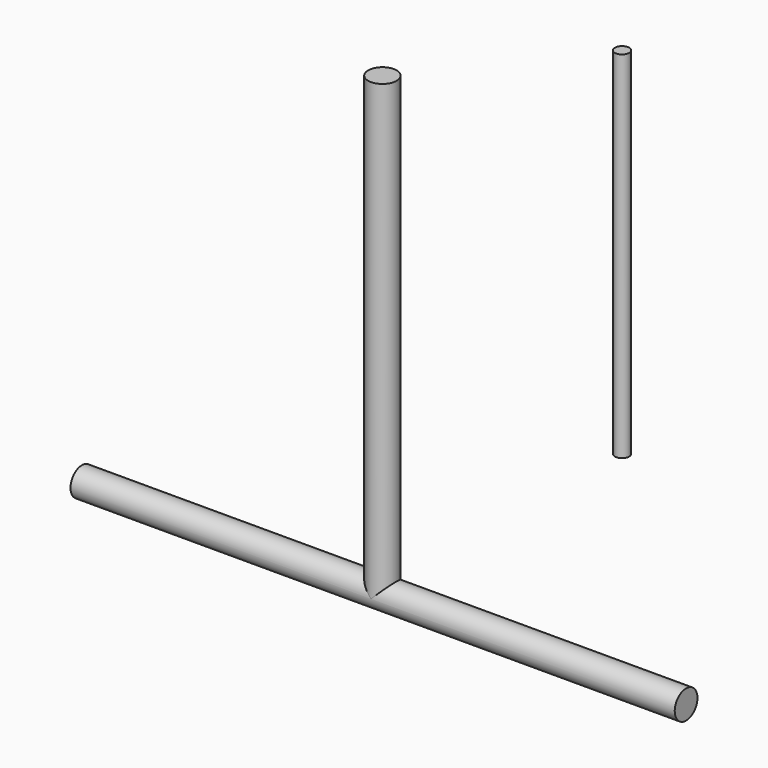
from build123d import *

# Parameters (mm, degrees)
F0_W     = 2.54
F0_H     = 81.28
F7_R     = 1.27
F8_DEPTH = 63.5


# Not quite as in the source:
# - the program builds the solid bodies; features that only make, move or delete a surface that nothing else refers to are left out


with BuildPart() as f1:
    # F0 (on Front) → F1 (revolve)
    with BuildSketch(Plane.XZ):
        with Locations((1.27, 0)):
            Rectangle(F0_W, F0_H)
    revolve(axis=Axis((0, 0, 0), (0, 0, -1)))

    # F4 (on face) → F5 (revolve)
    with BuildSketch(Plane.XZ):
        with BuildLine():
            Line((54.2592125952, -40.6373143196), (-51.1507874048, -40.6373143196))
            ThreePointArc((-51.1507874048, -40.6373143196), (-51.8947361806, -42.4333655438), (-53.6907874048, -43.1773143196))
            Line((-53.6907874048, -43.1773143196), (54.2592125952, -43.1773143196))
            Line((54.2592125952, -43.1773143196), (54.2592125952, -40.6373143196))
        make_face()
    revolve(axis=Axis((0.2842125952, 0, -40.6373143196), (1, 0, 0)))


with BuildPart() as f8:
    # F7 (on offset) → F8 (new body)
    with BuildSketch(Plane.XY.offset(-40.64)):
        with Locations((0, 53.5220466554)):
            Circle(F7_R)
    extrude(amount=F8_DEPTH)


solid = Compound([f1.part, f8.part])
